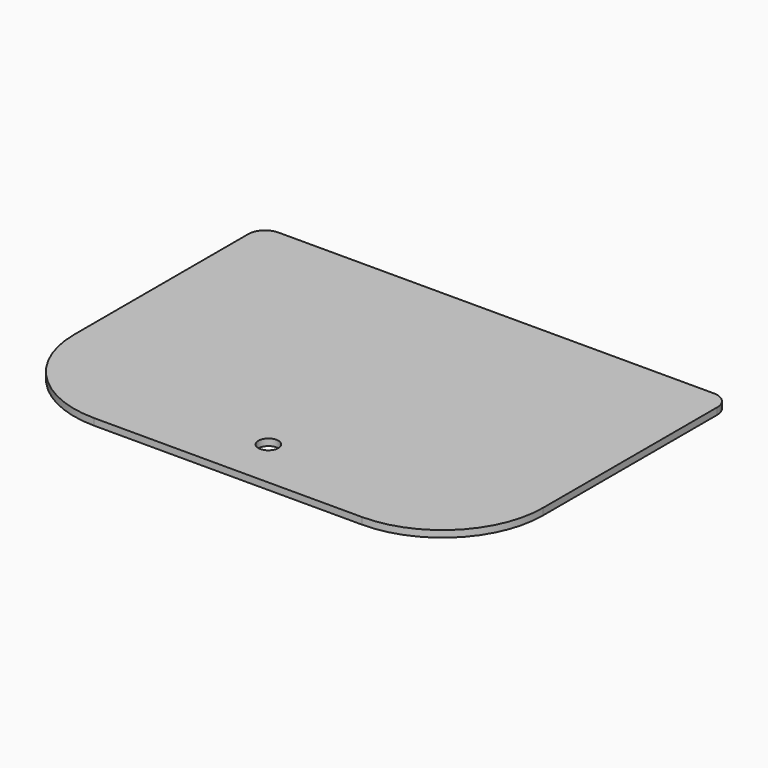
from build123d import *

# Parameters (mm, degrees)
F0_W     = 140
F0_H     = 100
F1_DEPTH = 2
F2_R     = 30
F3_R     = 3
F4_DEPTH = 25
F5_R     = 5


with BuildPart() as f1:
    # F0 (on Top) → F1 (new body)
    with BuildSketch(Plane.XY):
        Rectangle(F0_W, F0_H)
    extrude(amount=F1_DEPTH)

    # F2
    f2_edges = [f1.edges().sort_by_distance(p)[0] for p in [
        (-70, -50, 1),
        (70, -50, 1),
    ]]
    fillet(f2_edges, radius=F2_R)

    # F3 (on face) → F4 (cut)
    with BuildSketch(Plane.XY.offset(2)):
        with Locations((0, -35)):
            Circle(F3_R)
    extrude(amount=-F4_DEPTH, mode=Mode.SUBTRACT)

    # F5
    f5_edges = [f1.edges().sort_by_distance(p)[0] for p in [
        (70, 50, 1),
        (-70, 50, 1),
    ]]
    fillet(f5_edges, radius=F5_R)


solid = f1.part
